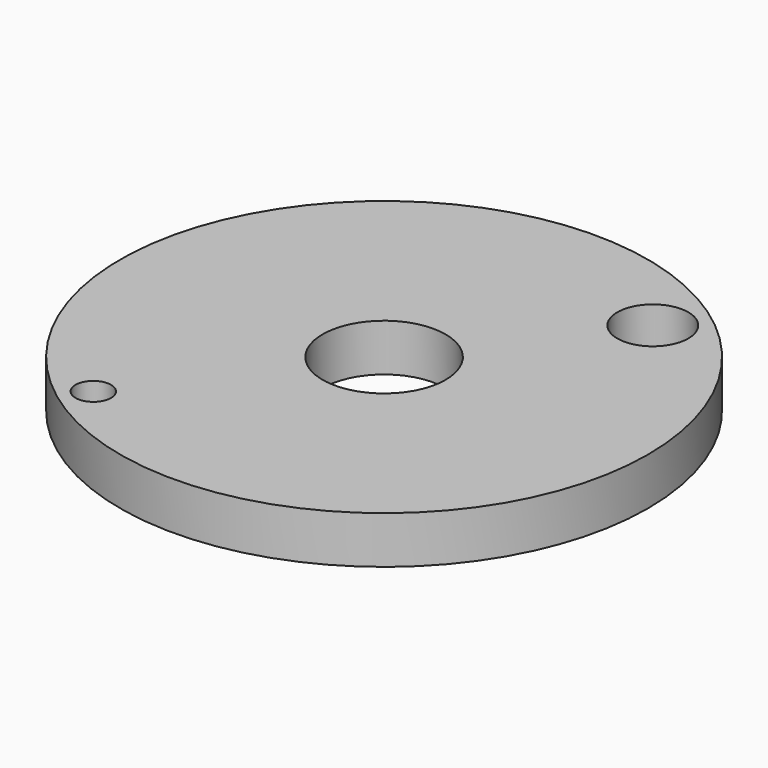
from build123d import *

# Parameters (mm, degrees)
F0_R     = 11.15
F1_DEPTH = 2
F2_R     = 1.5
F2_R_2   = 0.75
F2_R_3   = 2.6
F3_DEPTH = 25


# Not quite as in the source:
# - a feature names something its author has since deleted; it is built from what else it names


with BuildPart() as f1:
    # F0 (on Top) → F1 (new body)
    with BuildSketch(Plane.XY):
        Circle(F0_R)
    extrude(amount=F1_DEPTH)

    # F2 (on face) → F3 (cut)
    with BuildSketch(Plane.XY.offset(2)):
        with Locations((5.5076198523, 7.3067519161)):
            Circle(F2_R)
        with Locations((-5.9590641024, -7.9056660076)):
            Circle(F2_R_2)
        Circle(F2_R_3)
    extrude(amount=-F3_DEPTH, mode=Mode.SUBTRACT)


solid = f1.part
